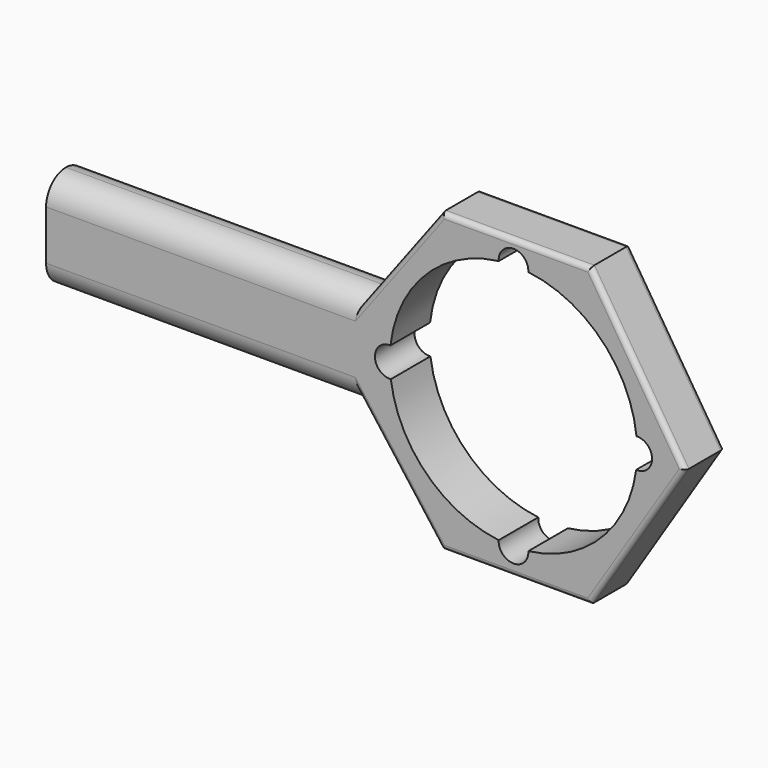
from build123d import *

# Parameters (mm, degrees)
F1_DEPTH = 10
F2_R     = 4.99999
F3_R     = 4.99999
F4_R     = 1
F5_R     = 1


# Not quite as in the source:
# - a fillet or chamfer is up to 0.001 mm smaller than in the source, because OpenCascade refuses the exact size


with BuildPart() as f1:
    # F0 (on Front) → F1 (new body)
    with BuildSketch(Plane.XZ):
        Polygon((0.5543106794, -10), (15.5543106794, -30), (45.5543106794, -30), (64.6686726809, 0), (45.5543106794, 30), (15.5543106794, 30), (0.5543106794, 10), (-64.4456893206, 10), (-64.4456893206, -10), align=None)
        with BuildLine():
            ThreePointArc((32.9945951312, 25.097839601), (47.7756292438, 17.8570035455), (54.8517478565, 2.9964106368))
            ThreePointArc((54.8517478565, 2.9964106368), (57.9982707821, -0.0333407521), (54.7851864872, -2.9924097466))
            ThreePointArc((54.7851864872, -2.9924097466), (47.5791639445, -17.4977896428), (32.9945951312, -24.542160399))
            ThreePointArc((32.9945951312, -24.542160399), (30, -27.722160399), (27.0054048688, -24.542160399))
            ThreePointArc((27.0054048688, -24.542160399), (12.4208360555, -17.4977896428), (5.2148135128, -2.9924097466))
            ThreePointArc((5.2148135128, -2.9924097466), (2.0017292179, -0.0333407521), (5.1482521435, 2.9964106368))
            ThreePointArc((5.1482521435, 2.9964106368), (12.2243707562, 17.8570035455), (27.0054048688, 25.097839601))
            ThreePointArc((27.0054048688, 25.097839601), (30, 28.277839601), (32.9945951312, 25.097839601))
        make_face(mode=Mode.SUBTRACT)
    extrude(amount=F1_DEPTH)

    # F2 (radius 5 in the source; OpenCascade refuses exactly that, so slightly less here)
    f2_edges = [f1.edges().sort_by_distance(p)[0] for p in [
        (-31.945689, -10, -10),
        (-31.945689, 0, -10),
    ]]
    fillet(f2_edges, radius=F2_R)

    # F3 (radius 5 in the source; OpenCascade refuses exactly that, so slightly less here)
    f3_edges = [f1.edges().sort_by_distance(p)[0] for p in [
        (-31.945689, 0, 10),
        (-31.945689, -10, 10),
    ]]
    fillet(f3_edges, radius=F3_R)

    # F4
    f4_edges = [f1.edges().sort_by_distance(p)[0] for p in [
        (8.054311, -10, 20),
        (30.554311, -10, 30),
        (55.111492, -10, 15),
        (55.111492, -10, -15),
        (30.554311, -10, -30),
        (8.054311, -10, -20),
    ]]
    fillet(f4_edges, radius=F4_R)

    # F5
    f5_edges = [f1.edges().sort_by_distance(p)[0] for p in [
        (30.554311, 0, 30),
        (55.111492, 0, 15),
        (55.111492, 0, -15),
        (30.554311, 0, -30),
        (8.054311, 0, -20),
        (8.054311, 0, 20),
    ]]
    fillet(f5_edges, radius=F5_R)


solid = f1.part
